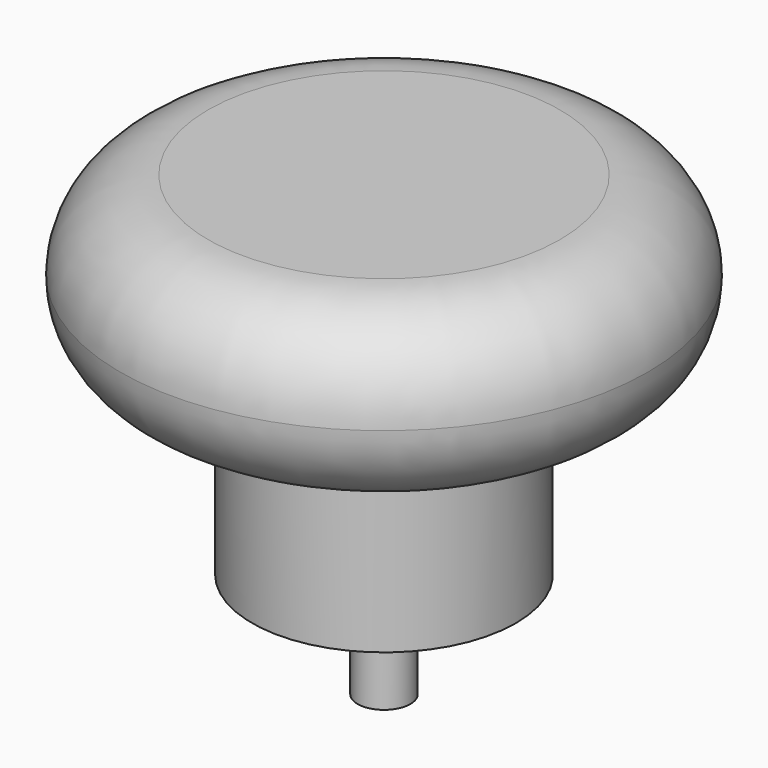
from build123d import *

# Parameters (mm, degrees)
F0_R     = 7.5
F0_R_2   = 1.5
F0_R_3   = 1
F1_DEPTH = 10
F2_DEPTH = 6
F3_R     = 15
F3_R_2   = 7.5
F4_DEPTH = 10
F5_R     = 4.99999


# Not quite as in the source:
# - a fillet or chamfer is up to 0.001 mm smaller than in the source, because OpenCascade refuses the exact size


with BuildPart() as f1:
    # F0 (on Top) → F1 (new body)
    with BuildSketch(Plane.XY):
        Circle(F0_R)
        Circle(F0_R_2, mode=Mode.SUBTRACT)
        Circle(F0_R_2)
        Circle(F0_R_3, mode=Mode.SUBTRACT)
        Circle(F0_R_3)
    extrude(amount=F1_DEPTH)

    # F0 (on Top) → F2 (join)
    with BuildSketch(Plane.XY):
        Circle(F0_R_2)
        Circle(F0_R_3, mode=Mode.SUBTRACT)
        Circle(F0_R_3)
    extrude(amount=-F2_DEPTH)

    # F3 (on face) → F4 (join)
    with BuildSketch(Plane.XY.offset(10)):
        Circle(F3_R)
        Circle(F3_R_2, mode=Mode.SUBTRACT)
        Circle(F3_R_2)
    extrude(amount=F4_DEPTH)

    # F5 (radius 5 in the source; OpenCascade refuses exactly that, so slightly less here)
    f5_edges = [f1.edges().sort_by_distance(p)[0] for p in [
        (15, 0, 15),
        (-15, 0, 10),
        (-15, 0, 20),
    ]]
    fillet(f5_edges, radius=F5_R)


solid = f1.part
